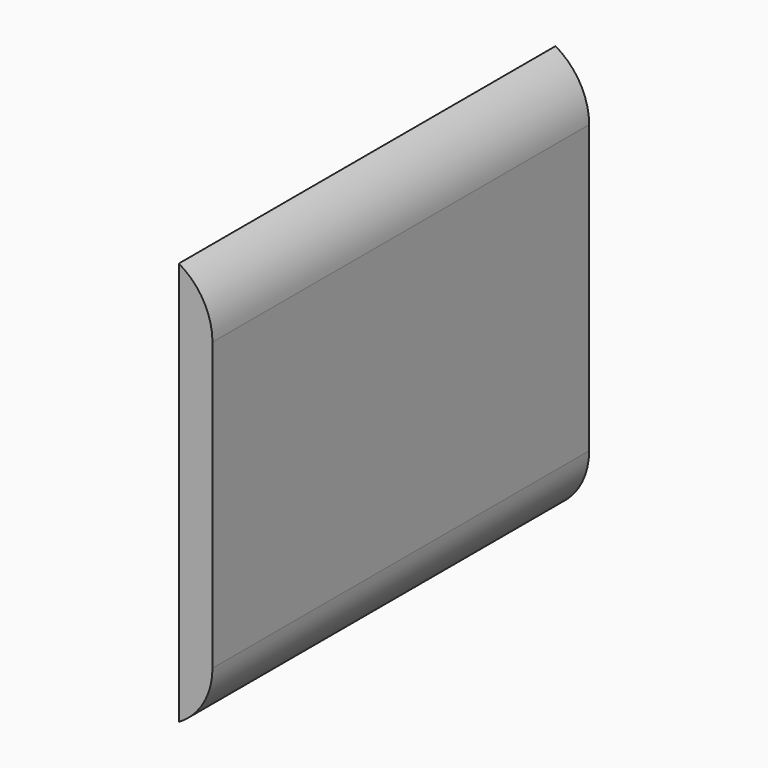
from build123d import *

# Parameters (mm, degrees)
F0_W        = 10
F0_H        = 120
F1_DEPTH    = 140
F2_T1_DEPTH = 226.6025403784


# Not quite as in the source:
# - a fillet or chamfer that OpenCascade refuses, or shapes differently, is made with other operations: its cross-section is extruded or revolved along the edge and cut away or added


with BuildPart() as f1:
    # F0 (on Front) → F1 (new body)
    with BuildSketch(Plane.XZ):
        Rectangle(F0_W, F0_H)
    extrude(amount=F1_DEPTH)

    # F2: fillet of radius 20 on 2 edges, made by hand

    # F2_s2 → F2_t1 (cut)
    with BuildSketch(Plane.XZ.offset(-43.3012701892)):
        with BuildLine():
            ThreePointArc((-5, 60), (2.3205080757, 52.6794919243), (5, 42.6794919243))
            Line((5, 42.6794919243), (5, 60))
            Line((5, 60), (-5, 60))
        make_face()
        with BuildLine():
            ThreePointArc((-5, -60), (2.3205080757, -52.6794919243), (5, -42.6794919243))
            Line((5, -42.6794919243), (5, -60))
            Line((5, -60), (-5, -60))
        make_face()
    extrude(amount=F2_T1_DEPTH, mode=Mode.SUBTRACT)


solid = f1.part
